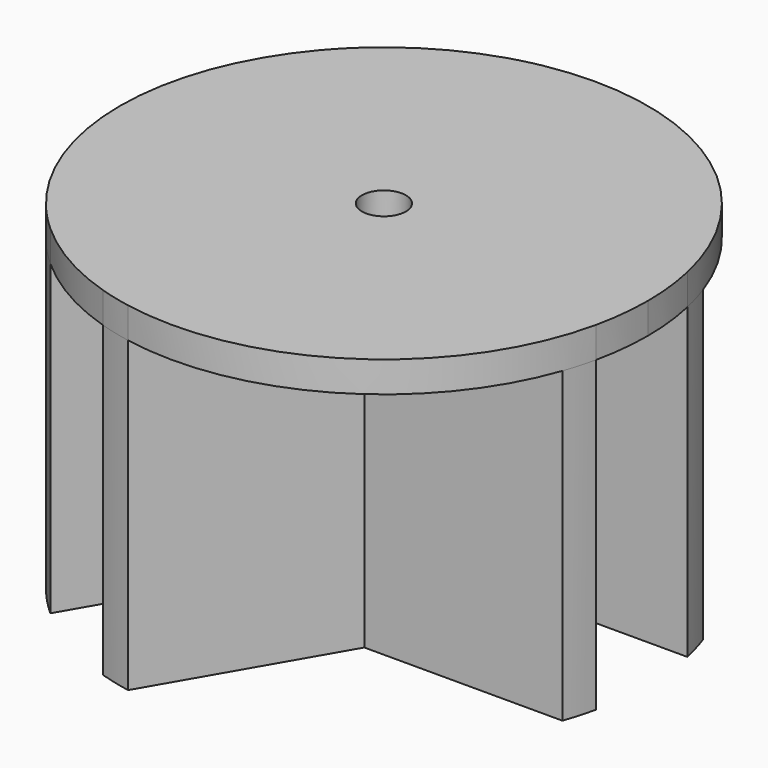
from build123d import *

# Parameters (mm, degrees)
F0_R     = 5
F1_DEPTH = 7
F2_DEPTH = 70


# Not quite as in the source:
# - after a boolean that leaves OpenCascade's solid faulty, fix() repairs it


with BuildPart() as f1:
    # F0 (on Top) → F1 (new body)
    with BuildSketch(Plane.XY):
        with BuildLine():
            Line((11.5470053838, 20), (56.5685424949, 20))
            ThreePointArc((56.5685424949, 20), (30, 51.9615242271), (-10.9637631718, 58.9897948557))
            Line((-10.9637631718, 58.9897948557), (11.5470053838, 20))
        make_face()
        with BuildLine():
            ThreePointArc((-10.9637631718, -58.9897948557), (30, -51.9615242271), (56.5685424949, -20))
            Line((56.5685424949, -20), (11.5470053838, -20))
            Line((11.5470053838, -20), (-10.9637631718, -58.9897948557))
        make_face()
        with BuildLine():
            ThreePointArc((58.5747385824, -13), (59.6426203103, -6.5389481208), (60, 0))
            ThreePointArc((60, 0), (59.6426203103, 6.5389481208), (58.5747385824, 13))
            Line((58.5747385824, 13), (15.5884572681, 13))
            Line((15.5884572681, 13), (7.5055534995, 13))
            Line((7.5055534995, 13), (11.2583302492, 6.5))
            ThreePointArc((11.2583302492, 6.5), (12.5570357418, 3.3646475863), (13, 0))
            ThreePointArc((13, 0), (12.5570357418, -3.3646475863), (11.2583302492, -6.5))
            Line((11.2583302492, -6.5), (7.5055534995, -13))
            Line((7.5055534995, -13), (15.5884572681, -13))
            Line((15.5884572681, -13), (58.5747385824, -13))
        make_face()
        with BuildLine():
            ThreePointArc((56.5685424949, -20), (57.6779316057, -16.5304629604), (58.5747385824, -13))
            Line((58.5747385824, -13), (15.5884572681, -13))
            Line((15.5884572681, -13), (11.5470053838, -20))
            Line((11.5470053838, -20), (56.5685424949, -20))
        make_face()
        with BuildLine():
            Line((15.5884572681, 13), (58.5747385824, 13))
            ThreePointArc((58.5747385824, 13), (57.6779316057, 16.5304629604), (56.5685424949, 20))
            Line((56.5685424949, 20), (11.5470053838, 20))
            Line((11.5470053838, 20), (15.5884572681, 13))
        make_face()
        with BuildLine():
            Line((3.4641016151, -20), (7.5055534995, -13))
            Line((7.5055534995, -13), (0, -13))
            ThreePointArc((0, -13), (-6.6785653008, -11.1533297953), (-11.4597294399, -6.1379639265))
            Line((-11.4597294399, -6.1379639265), (-14.736550409, -0.4623435209))
            Line((-14.736550409, -0.4623435209), (-18.7780022933, -7.4623435209))
            Line((-18.7780022933, -7.4623435209), (-40.1906368837, -44.5501145553))
            ThreePointArc((-40.1906368837, -44.5501145553), (-29.7919429343, -52.081091926), (-18.029039042, -57.2272116324))
            Line((-18.029039042, -57.2272116324), (3.4641016151, -20))
        make_face()
        with BuildLine():
            Line((-14.736550409, -0.4623435209), (-40.5407150531, 44.2317806897))
            ThreePointArc((-40.5407150531, 44.2317806897), (-43.1499853268, 41.6902718424), (-45.6002292233, 38.995116294))
            Line((-45.6002292233, 38.995116294), (-23.0863883339, 0))
            Line((-23.0863883339, 0), (-18.7780022933, -7.4623435209))
            Line((-18.7780022933, -7.4623435209), (-14.736550409, -0.4623435209))
        make_face()
        with BuildLine():
            Line((0, 13), (7.5055534995, 13))
            Line((7.5055534995, 13), (3.4641016151, 20))
            Line((3.4641016151, 20), (-18.029039042, 57.2272116324))
            ThreePointArc((-18.029039042, 57.2272116324), (-29.9970720244, 51.9632145846), (-40.5407150531, 44.2317806897))
            Line((-40.5407150531, 44.2317806897), (-14.736550409, -0.4623435209))
            Line((-14.736550409, -0.4623435209), (-12.5822883529, 3.2689478131))
            ThreePointArc((-12.5822883529, 3.2689478131), (-11.2583302492, 6.5), (-9.1221360262, 9.2621074448))
            ThreePointArc((-9.1221360262, 9.2621074448), (-4.9291278751, 12.0292850324), (0, 13))
        make_face()
        with BuildLine():
            Line((-23.0863883339, 0), (-45.6002292233, 38.995116294))
            ThreePointArc((-45.6002292233, 38.995116294), (-60, 0), (-45.6002292233, -38.995116294))
            Line((-45.6002292233, -38.995116294), (-23.0863883339, 0))
        make_face()
        with BuildLine():
            Line((11.5470053838, 20), (-10.9637631718, 58.9897948557))
            ThreePointArc((-10.9637631718, 58.9897948557), (-14.5231649428, 58.2157854885), (-18.029039042, 57.2272116324))
            Line((-18.029039042, 57.2272116324), (3.4641016151, 20))
            Line((3.4641016151, 20), (11.5470053838, 20))
        make_face()
        with BuildLine():
            ThreePointArc((-45.6002292233, -38.995116294), (-42.9852611748, -41.8600922328), (-40.1906368837, -44.5501145553))
            Line((-40.1906368837, -44.5501145553), (-18.7780022933, -7.4623435209))
            Line((-18.7780022933, -7.4623435209), (-23.0863883339, 0))
            Line((-23.0863883339, 0), (-45.6002292233, -38.995116294))
        make_face()
        with BuildLine():
            ThreePointArc((-18.029039042, -57.2272116324), (-14.5231649428, -58.2157854885), (-10.9637631718, -58.9897948557))
            Line((-10.9637631718, -58.9897948557), (11.5470053838, -20))
            Line((11.5470053838, -20), (3.4641016151, -20))
            Line((3.4641016151, -20), (-18.029039042, -57.2272116324))
        make_face()
        Polygon((11.5470053838, -20), (15.5884572681, -13), (7.5055534995, -13), (3.4641016151, -20), align=None)
        Polygon((7.5055534995, 13), (15.5884572681, 13), (11.5470053838, 20), (3.4641016151, 20), align=None)
        with BuildLine():
            Line((0, -13), (7.5055534995, -13))
            Line((7.5055534995, -13), (11.2583302492, -6.5))
            ThreePointArc((11.2583302492, -6.5), (6.5, -11.2583302492), (0, -13))
        make_face()
        with BuildLine():
            Line((-12.5822883529, 3.2689478131), (-9.1221360262, 9.2621074448))
            ThreePointArc((-9.1221360262, 9.2621074448), (-11.2583302492, 6.5), (-12.5822883529, 3.2689478131))
        make_face()
        with BuildLine():
            Line((11.2583302492, 6.5), (7.5055534995, 13))
            Line((7.5055534995, 13), (0, 13))
            ThreePointArc((0, 13), (6.5, 11.2583302492), (11.2583302492, 6.5))
        make_face()
        with BuildLine():
            Line((-14.736550409, -0.4623435209), (-11.4597294399, -6.1379639265))
            ThreePointArc((-11.4597294399, -6.1379639265), (-12.9084140005, -1.5404051392), (-12.5822883529, 3.2689478131))
            Line((-12.5822883529, 3.2689478131), (-14.736550409, -0.4623435209))
        make_face()
        with BuildLine():
            ThreePointArc((11.2583302492, 6.5), (6.5, 11.2583302492), (0, 13))
            ThreePointArc((0, 13), (-4.9291278751, 12.0292850324), (-9.1221360262, 9.2621074448))
            Line((-9.1221360262, 9.2621074448), (-12.5822883529, 3.2689478131))
            ThreePointArc((-12.5822883529, 3.2689478131), (-12.9084140005, -1.5404051392), (-11.4597294399, -6.1379639265))
            ThreePointArc((-11.4597294399, -6.1379639265), (-6.6785653008, -11.1533297953), (0, -13))
            ThreePointArc((0, -13), (6.5, -11.2583302492), (11.2583302492, -6.5))
            ThreePointArc((11.2583302492, -6.5), (12.5570357418, -3.3646475863), (13, 0))
            ThreePointArc((13, 0), (12.5570357418, 3.3646475863), (11.2583302492, 6.5))
        make_face()
        Circle(F0_R, mode=Mode.SUBTRACT)
    extrude(amount=F1_DEPTH)

    # F0 (on Top) → F2 (join)
    with BuildSketch(Plane.XY):
        with BuildLine():
            ThreePointArc((56.5685424949, -20), (57.6779316057, -16.5304629604), (58.5747385824, -13))
            Line((58.5747385824, -13), (15.5884572681, -13))
            Line((15.5884572681, -13), (11.5470053838, -20))
            Line((11.5470053838, -20), (56.5685424949, -20))
        make_face()
        Polygon((11.5470053838, -20), (15.5884572681, -13), (7.5055534995, -13), (3.4641016151, -20), align=None)
        with BuildLine():
            ThreePointArc((-18.029039042, -57.2272116324), (-14.5231649428, -58.2157854885), (-10.9637631718, -58.9897948557))
            Line((-10.9637631718, -58.9897948557), (11.5470053838, -20))
            Line((11.5470053838, -20), (3.4641016151, -20))
            Line((3.4641016151, -20), (-18.029039042, -57.2272116324))
        make_face()
        with BuildLine():
            ThreePointArc((-45.6002292233, -38.995116294), (-42.9852611748, -41.8600922328), (-40.1906368837, -44.5501145553))
            Line((-40.1906368837, -44.5501145553), (-18.7780022933, -7.4623435209))
            Line((-18.7780022933, -7.4623435209), (-23.0863883339, 0))
            Line((-23.0863883339, 0), (-45.6002292233, -38.995116294))
        make_face()
        with BuildLine():
            Line((-14.736550409, -0.4623435209), (-40.5407150531, 44.2317806897))
            ThreePointArc((-40.5407150531, 44.2317806897), (-43.1499853268, 41.6902718424), (-45.6002292233, 38.995116294))
            Line((-45.6002292233, 38.995116294), (-23.0863883339, 0))
            Line((-23.0863883339, 0), (-18.7780022933, -7.4623435209))
            Line((-18.7780022933, -7.4623435209), (-14.736550409, -0.4623435209))
        make_face()
        with BuildLine():
            Line((11.5470053838, 20), (-10.9637631718, 58.9897948557))
            ThreePointArc((-10.9637631718, 58.9897948557), (-14.5231649428, 58.2157854885), (-18.029039042, 57.2272116324))
            Line((-18.029039042, 57.2272116324), (3.4641016151, 20))
            Line((3.4641016151, 20), (11.5470053838, 20))
        make_face()
        Polygon((7.5055534995, 13), (15.5884572681, 13), (11.5470053838, 20), (3.4641016151, 20), align=None)
        with BuildLine():
            Line((15.5884572681, 13), (58.5747385824, 13))
            ThreePointArc((58.5747385824, 13), (57.6779316057, 16.5304629604), (56.5685424949, 20))
            Line((56.5685424949, 20), (11.5470053838, 20))
            Line((11.5470053838, 20), (15.5884572681, 13))
        make_face()
        with BuildLine():
            ThreePointArc((11.2583302492, 6.5), (6.5, 11.2583302492), (0, 13))
            ThreePointArc((0, 13), (-4.9291278751, 12.0292850324), (-9.1221360262, 9.2621074448))
            Line((-9.1221360262, 9.2621074448), (-12.5822883529, 3.2689478131))
            ThreePointArc((-12.5822883529, 3.2689478131), (-12.9084140005, -1.5404051392), (-11.4597294399, -6.1379639265))
            ThreePointArc((-11.4597294399, -6.1379639265), (-6.6785653008, -11.1533297953), (0, -13))
            ThreePointArc((0, -13), (6.5, -11.2583302492), (11.2583302492, -6.5))
            ThreePointArc((11.2583302492, -6.5), (12.5570357418, -3.3646475863), (13, 0))
            ThreePointArc((13, 0), (12.5570357418, 3.3646475863), (11.2583302492, 6.5))
        make_face()
        Circle(F0_R, mode=Mode.SUBTRACT)
    extrude(amount=-F2_DEPTH)

    add(f1.part.fix(), mode=Mode.REPLACE)


solid = f1.part
